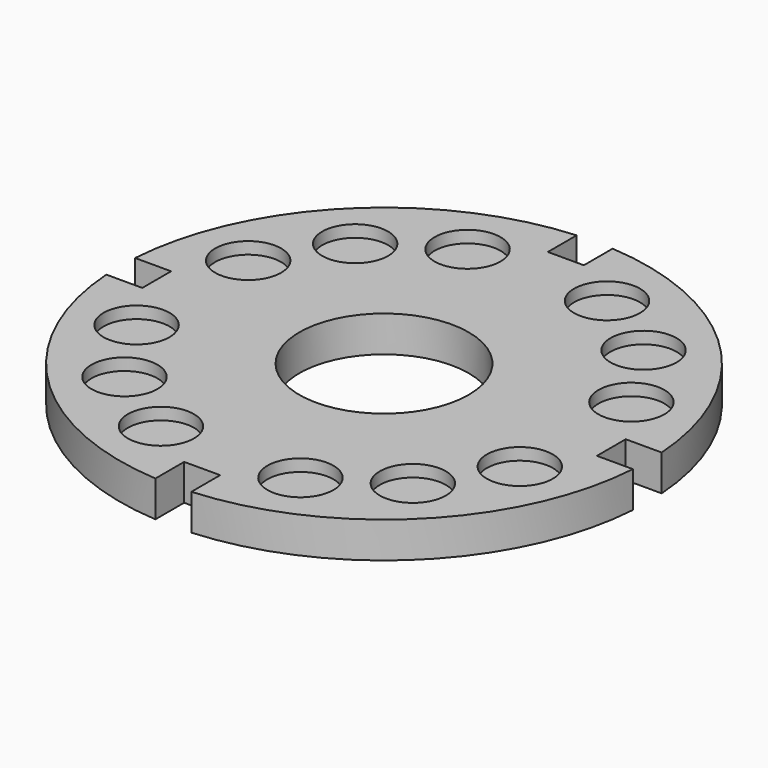
from build123d import *

# Parameters (mm, degrees)
F0_R            = 44.8437
F0_R_2          = 17.4625
F0_W            = 19.05
F0_H            = 6.35
F1_DEPTH        = 19.05
F2_DEPTH        = 6.35
F2_COPIES_COUNT = 4
F3_DEPTH        = 19.051
F3_COPIES_COUNT = 4
F5_DEPTH        = 25.4


# Not quite as in the source:
# - a pattern or mirror of a feature is missing from the dataset's text; its kind, count and spacing are read off the source's solid


with BuildPart() as f1:
    # F0 (on Top) → F1 (new body)
    with BuildSketch(Plane.XY):
        with BuildLine():
            ThreePointArc((-9.525, 139.3749058296), (-95.3557746023, -102.0948884617), (139.7, 0))
            ThreePointArc((139.7, 0), (102.0948884617, 95.3557746023), (9.525, 139.3749058296))
            Line((9.525, 139.3749058296), (9.525, 120.3249058296))
            Line((9.525, 120.3249058296), (9.525, 113.9749058296))
            Line((9.525, 113.9749058296), (-9.525, 113.9749058296))
            Line((-9.525, 113.9749058296), (-9.525, 120.3249058296))
            Line((-9.525, 120.3249058296), (-9.525, 139.3749058296))
        make_face()
        Circle(F0_R, mode=Mode.SUBTRACT)
        with Locations((101.4398184138, 36.921074472)):
            Circle(F0_R_2, mode=Mode.SUBTRACT)
        with Locations((36.921074472, 101.4398184138)):
            Circle(F0_R_2, mode=Mode.SUBTRACT)
        with Locations((76.3321770291, 76.3321770291)):
            Circle(F0_R_2, mode=Mode.SUBTRACT)
        with BuildLine():
            Line((9.525, 120.3249058296), (9.525, 139.3749058296))
            ThreePointArc((9.525, 139.3749058296), (0, 139.7), (-9.525, 139.3749058296))
            Line((-9.525, 139.3749058296), (-9.525, 120.3249058296))
            Line((-9.525, 120.3249058296), (9.525, 120.3249058296))
        make_face()
        with Locations((36.921074472, 101.4398184138)):
            Circle(F0_R_2)
        with Locations((76.3321770291, 76.3321770291)):
            Circle(F0_R_2)
        with Locations((101.4398184138, 36.921074472)):
            Circle(F0_R_2)
        with Locations((0, 117.1499058296)):
            Rectangle(F0_W, F0_H)
        Circle(F0_R)
    extrude(amount=-F1_DEPTH)

    # F0 (on Top) → F2 (cut)
    with BuildSketch(Plane.XY):
        with Locations((36.921074472, 101.4398184138)):
            Circle(F0_R_2)
        with Locations((76.3321770291, 76.3321770291)):
            Circle(F0_R_2)
        with Locations((101.4398184138, 36.921074472)):
            Circle(F0_R_2)
    f2 = extrude(amount=-F2_DEPTH, mode=Mode.SUBTRACT)

    # F2_copies: F2 ×4 about axis
    f2_copies_axis = Axis((0, 0, 0), (0, 0, 1))
    for i in range(1, F2_COPIES_COUNT):
        add(f2.rotate(f2_copies_axis, i * 360 / F2_COPIES_COUNT), mode=Mode.SUBTRACT)

    # F0 (on Top) → F3 (cut, through all)
    with BuildSketch(Plane.XY):
        with BuildLine():
            Line((9.525, 120.3249058296), (9.525, 139.3749058296))
            ThreePointArc((9.525, 139.3749058296), (0, 139.7), (-9.525, 139.3749058296))
            Line((-9.525, 139.3749058296), (-9.525, 120.3249058296))
            Line((-9.525, 120.3249058296), (9.525, 120.3249058296))
        make_face()
    f3 = extrude(amount=-F3_DEPTH, mode=Mode.SUBTRACT)

    # F3_copies: F3 ×4 about axis
    f3_copies_axis = Axis((0, 0, 0), (0, 0, 1))
    for i in range(1, F3_COPIES_COUNT):
        add(f3.rotate(f3_copies_axis, i * 360 / F3_COPIES_COUNT), mode=Mode.SUBTRACT)

    # F0 (on Top) → F5 (cut)
    with BuildSketch(Plane.XY):
        Circle(F0_R)
    extrude(amount=-F5_DEPTH, mode=Mode.SUBTRACT)


solid = f1.part
